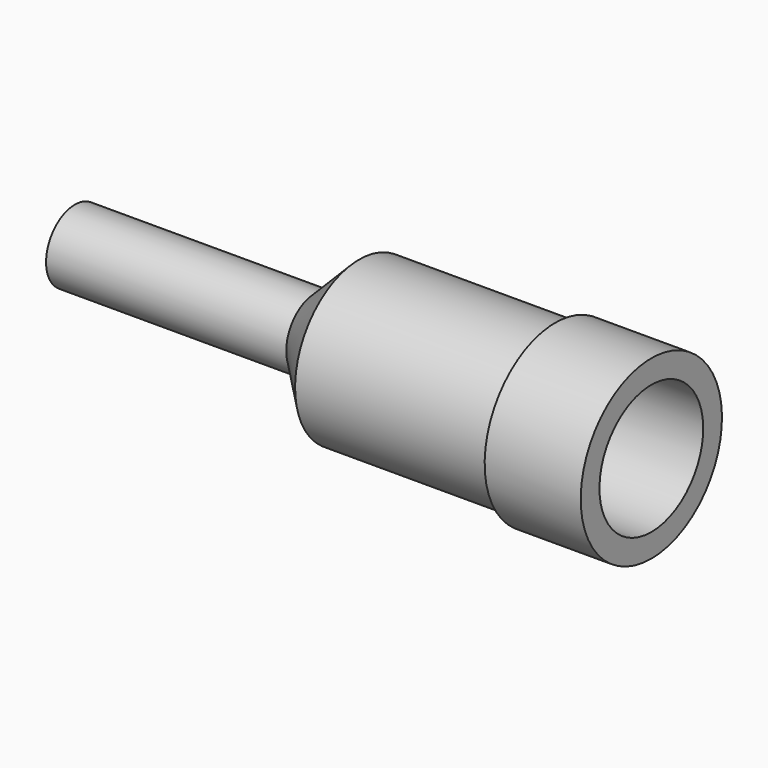
from build123d import *

# Parameters (mm, degrees)
F2_S5_R     = 8.4836
F2_T6_DEPTH = 14


# Not quite as in the source:
# - a fillet or chamfer that OpenCascade refuses, or shapes differently, is made with other operations: its cross-section is extruded or revolved along the edge and cut away or added


with BuildPart() as f1:
    # F0 (on Front) → F1 (revolve)
    with BuildSketch(Plane.XZ):
        Polygon((-33.02, 0), (-2.54, 0), (-2.54, -4.6736), (17.78, -4.6736), (17.78, -5.5245), (27.94, -5.5245), (27.94, -3.048), (0, -3.048), (0, 2.921), (-33.02, 2.921), align=None)
    revolve(axis=Axis((-5.3856544969, 0, 3.81), (1, 0, 0)))

    # F2: chamfer of 5.08 on 1 edges, made by hand


with BuildPart() as f2_tool2:
    # F2_s3 → F2_t4 (revolve)
    with BuildSketch(Plane.XZ):
        Polygon((-7.62, 0), (-2.54, -5.08), (-2.54, 0), align=None)
    revolve(axis=Axis((-2.54, 0, 3.81), (1, 0, 0)))

    # F2_s5 → F2_t6 (intersect, symmetric)
    with BuildSketch(Plane.YZ.offset(-5.1)):
        with Locations((0, 3.81)):
            Circle(F2_S5_R)
    extrude(amount=F2_T6_DEPTH, both=True, mode=Mode.INTERSECT)


with BuildPart() as f1_1:
    add(f1.part)

    # F2_t1: union F2_tool2
    add(f2_tool2.part)


solid = f1_1.part
